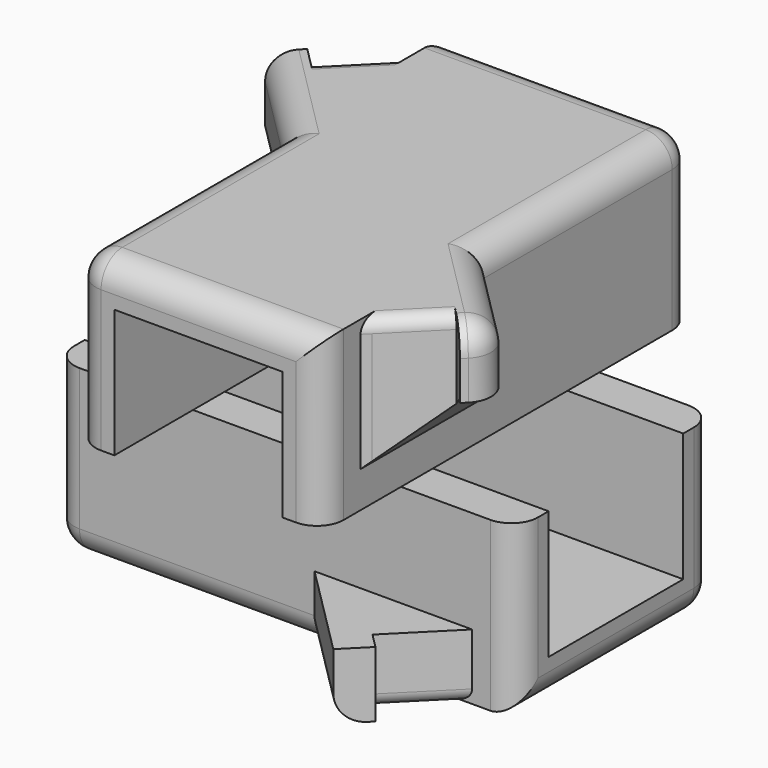
from build123d import *

# Parameters (mm, degrees)
F0_W        = 18.7
F0_H        = 18.7
F0_W_2      = 12.7
F0_H_2      = 12.7
F1_DEPTH    = 17.5
F2_W        = 41.0629063845
F2_H        = 23.0880221352
F3_DEPTH    = 19.9
F5_START    = 4.4
F5_DEPTH    = 4.95
F6_T4_DEPTH = 8.1847385173
F6_T9_DEPTH = 8.4077243134
F7_DEPTH    = 25
F8_SIZE     = 5
F9_R        = 2
F11_ANGLE   = 90
F13_ANGLE   = 180


# Not quite as in the source:
# - a fillet or chamfer that OpenCascade refuses, or shapes differently, is made with other operations: its cross-section is extruded or revolved along the edge and cut away or added


with BuildPart() as f1:
    # F0 (on Front) → F1 (new body, symmetric)
    with BuildSketch(Plane.XZ):
        Rectangle(F0_W, F0_H)
        Rectangle(F0_W_2, F0_H_2, mode=Mode.SUBTRACT)
    extrude(amount=F1_DEPTH, both=True)

    # F2 (on Front) → F3 (cut, symmetric)
    with BuildSketch(Plane.XZ):
        with Locations((0, -14.8746278137)):
            Rectangle(F2_W, F2_H)
    extrude(amount=F3_DEPTH, both=True, mode=Mode.SUBTRACT)

    # F4 (on Top) → F5 (join)
    with BuildSketch(Plane.XY.offset(F5_START)):
        Polygon((-13.5273919234, 9.9516930848), (-14.6533008589, 11.0776020203), (-16.4210678119, 9.3098350673), (8.066416296, -15.1776490405), (9.8341832489, -13.4098820875), (13.3697171549, -9.8743481816), (14.6519559955, -11.1565870222), (16.4197229484, -9.3888200692), (-8.2240910645, 15.2549939437), (-9.9918580175, 13.4872269907), align=None)
    extrude(amount=F5_DEPTH)

    # F6: fillet of radius 1 on 2 edges, made by hand


with BuildPart() as f6_tool2:
    # F6_s3 → F6_t4 (new body)
    with BuildSketch(Plane(origin=(1.7476844866, 1.7476844866, 0), x_dir=(0, 0, 1), z_dir=(-0.7071067812, -0.7071067812, 0))):
        with BuildLine():
            ThreePointArc((9.35, -15.4360362217), (9.0571067812, -16.1431430029), (8.35, -16.4360362217))
            Line((8.35, -16.4360362217), (9.35, -16.4360362217))
            Line((9.35, -16.4360362217), (9.35, -15.4360362217))
        make_face()
    extrude(amount=F6_T4_DEPTH)

    split(bisect_by=Plane.YZ.offset(9.35), keep=Keep.TOP)


with BuildPart() as f1_1:
    add(f1.part)

    # F6_t1: cut F6_tool2
    add(f6_tool2.part, mode=Mode.SUBTRACT)


with BuildPart() as f6_tool7:
    # F6_s8 → F6_t9 (new body)
    with BuildSketch(Plane(origin=(-1.7878494193, -1.7878494193, 0), x_dir=(0, 0, 1), z_dir=(0.7071067812, 0.7071067812, 0))):
        with BuildLine():
            ThreePointArc((9.35, -15.6022202254), (9.0571067812, -16.3093270066), (8.35, -16.6022202254))
            Line((8.35, -16.6022202254), (9.35, -16.6022202254))
            Line((9.35, -16.6022202254), (9.35, -15.6022202254))
        make_face()
    extrude(amount=F6_T9_DEPTH)

    split(bisect_by=Plane.YZ.offset(-9.35), keep=Keep.BOTTOM)


with BuildPart() as f1_2:
    add(f1_1.part)

    # F6_t6: cut F6_tool7
    add(f6_tool7.part, mode=Mode.SUBTRACT)

    # F0 (on Front) → F7 (cut, symmetric)
    with BuildSketch(Plane.XZ):
        Rectangle(F0_W_2, F0_H_2)
    extrude(amount=F7_DEPTH, both=True, mode=Mode.SUBTRACT)

    # F8
    f8_edges = [f1_2.edges().sort_by_distance(p)[0] for p in [
        (9.35, -8.106581, 4.4),
    ]]
    chamfer(f8_edges, length=F8_SIZE)

    # F9
    f9_edges = [f1_2.edges().sort_by_distance(p)[0] for p in [
        (9.35, 7.590451, 9.35),
        (-9.35, -7.630616, 9.35),
        (0, -17.5, 9.35),
        (0, 17.5, 9.35),
        (16.419723, -9.38882, 6.875),
        (12.884861, -5.853959, 9.35),
        (-12.885534, 5.774301, 9.35),
        (15.535839, -10.272704, 9.35),
        (9.35, -17.5, 3.009692),
        (-9.35, -17.5, 3.009692),
        (9.35, 17.5, 3.009692),
        (-9.35, 17.5, 3.009692),
    ]]
    fillet(f9_edges, radius=F9_R)


with BuildPart() as f10_1:
    # F10: copy of F1
    add(f1_2.part.moved(Location((0, 0, -15.6))))


with BuildPart() as f10_1_1:
    # F11: moved
    add(f10_1.part.rotate(Axis((0, 0, 16.1133408546), (0, 0, 1)), F11_ANGLE))


with BuildPart() as f10_1_2:
    # F13: moved
    add(f10_1_1.part.rotate(Axis((0, 0.7898686454, -11.3741233945), (0, 1, 0)), F13_ANGLE))


solid = Compound([f1_2.part, f10_1_2.part])
